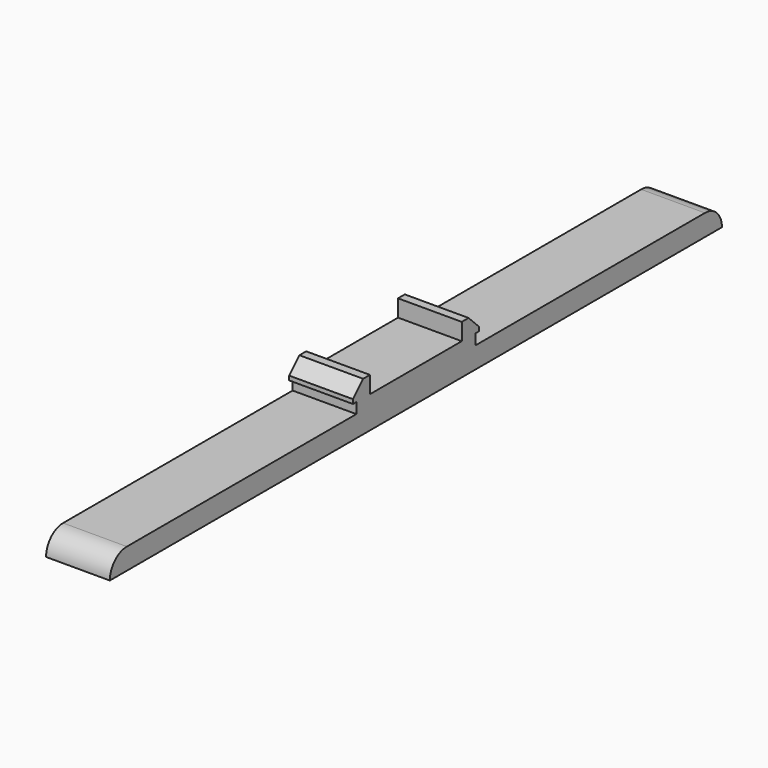
from build123d import *

# Parameters (mm, degrees)
F1_DEPTH = 15
F2_SIZE  = 3
F3_R     = 4.99999


# Not quite as in the source:
# - a fillet or chamfer is up to 0.001 mm smaller than in the source, because OpenCascade refuses the exact size


with BuildPart() as f1:
    # F0 (on Right) → F1 (new body)
    with BuildSketch(Plane.YZ):
        Polygon((13.5, 7.5), (17.5, 7.5), (18.5, 7.5), (18.5, 11.5), (13.5, 11.5), align=None)
        Polygon((-17.5, 5), (17.5, 5), (17.5, 7.5), (13.5, 7.5), (-13.5, 7.5), (-17.5, 7.5), align=None)
        Polygon((90, 0), (90, 5), (17.5, 5), (-17.5, 5), (-90, 5), (-90, 0), align=None)
        Polygon((-18.5, 7.5), (-17.5, 7.5), (-13.5, 7.5), (-13.5, 11.5), (-18.5, 11.5), align=None)
    extrude(amount=F1_DEPTH)

    # F2
    f2_edges = [f1.edges().sort_by_distance(p)[0] for p in [
        (7.5, -18.5, 11.5),
        (7.5, 18.5, 11.5),
    ]]
    chamfer(f2_edges, length=F2_SIZE)

    # F3 (radius 5 in the source; OpenCascade refuses exactly that, so slightly less here)
    f3_edges = [f1.edges().sort_by_distance(p)[0] for p in [
        (7.5, 90, 5),
        (7.5, -90, 5),
    ]]
    fillet(f3_edges, radius=F3_R)


solid = f1.part
